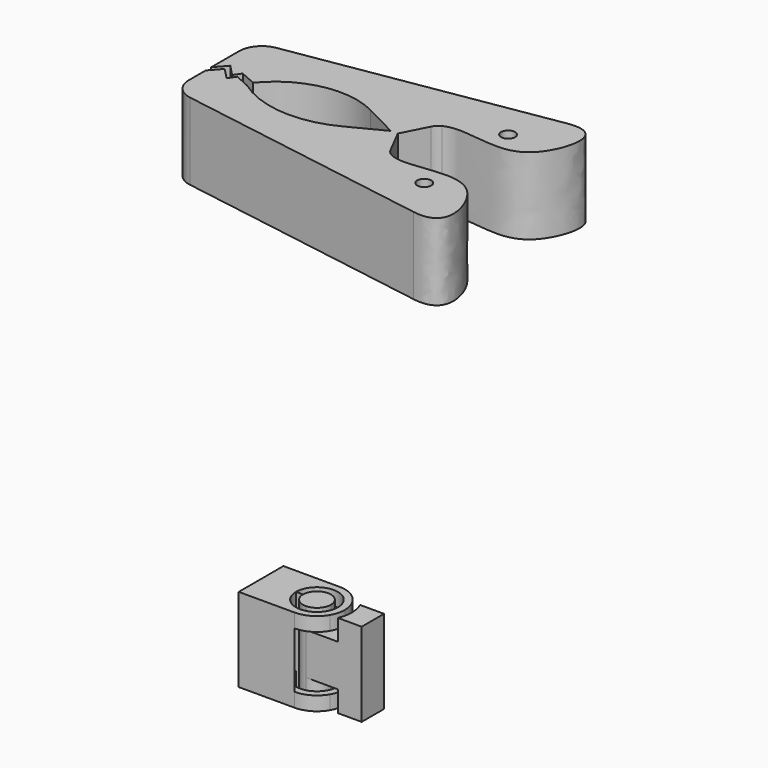
from build123d import *

# Parameters (mm, degrees)
F0_R     = 1
F1_DEPTH = 11
F3_DEPTH = 6
F4_DEPTH = 4
F5_DEPTH = 3
F6_DEPTH = 6


# Not quite as in the source:
# - a feature names something its author has since deleted; it is built from what else it names


with BuildPart() as f1:
    # F0 (on Top) → F1 (new body)
    with BuildSketch(Plane.XY):
        with BuildLine():
            Line((-56.5394303022, 63.5646519078), (-56.5394303022, 60.5646519078))
            Line((-56.5394303022, 60.5646519078), (-56.5394303022, 58.5646519078))
            Line((-56.5394303022, 58.5646519078), (-55.1112962965, 60.1865433678))
            Line((-55.1112962965, 60.1865433678), (-53.5394303022, 58.5646519078))
            Line((-53.5394303022, 58.5646519078), (-52.8413255975, 59.585552632))
            Line((-52.8413255975, 59.585552632), (-50.5394303022, 58.5646519078))
            ThreePointArc((-50.5394303022, 58.5646519078), (-43.8778670045, 62.6266002152), (-36.1451600741, 61.5868439218))
            Line((-36.1451600741, 61.5868439218), (-31.2319873402, 59.0646519078))
            Line((-31.2319873402, 59.0646519078), (-36.1451600741, 56.5424598938))
            ThreePointArc((-36.1451600741, 56.5424598938), (-43.5460973086, 55.0399418647), (-50.6461998164, 57.612873414))
            Line((-50.6461998164, 57.612873414), (-52.831540008, 58.5998629716))
            Line((-52.831540008, 58.5998629716), (-53.5394303022, 57.5646519078))
            Line((-53.5394303022, 57.5646519078), (-55.1112962965, 59.1865433678))
            Line((-55.1112962965, 59.1865433678), (-56.5394303022, 57.5646519078))
            Line((-56.5394303022, 57.5646519078), (-56.5394303022, 54.5646519078))
            ThreePointArc((-56.5394303022, 54.5646519078), (-55.7660672354, 52.4605684374), (-53.8141510367, 51.3581706702))
            Line((-53.8141510367, 51.3581706702), (-17.0027786636, 45.3461106944))
            add(Edge.make_bspline(
                [(-27.5149940739, 54.5646519078), (-25.8077646027, 53.6646211006), (-20.1492133777, 55.1651591419), (-13.9447941806, 53.7805000119), (-11.9302922568, 44.5176685435), (-17.0027786636, 45.3461106944)],
                knots=[0, 0, 0, 0, 0.3389884786, 0.6657804562, 1, 1, 1, 1], degree=3))
            ThreePointArc((-27.5149940739, 54.5646519078), (-28.0042315995, 54.9274057779), (-28.3616043344, 55.4205877474))
            Line((-28.3616043344, 55.4205877474), (-30.2319873402, 59.0646519078))
            Line((-30.2319873402, 59.0646519078), (-28.3616043344, 62.7087160682))
            ThreePointArc((-28.3616043344, 62.7087160682), (-28.0042315995, 63.2018980376), (-27.5149940739, 63.5646519078))
            add(Edge.make_bspline(
                [(-27.5149940739, 63.5646519078), (-25.8077646027, 64.464682715), (-20.1492133777, 62.9641446737), (-13.9447941806, 64.3488038037), (-11.9302922568, 73.6116352721), (-17.0027786636, 72.7831931212)],
                knots=[0, 0, 0, 0, 0.3389884786, 0.6657804562, 1, 1, 1, 1], degree=3))
            Line((-17.0027786636, 72.7831931212), (-53.8141510367, 66.7711331454))
            ThreePointArc((-53.8141510367, 66.7711331454), (-55.7660672354, 65.6687353782), (-56.5394303022, 63.5646519078))
        make_face()
        with Locations((-20.4416182045, 51.5646519078)):
            Circle(F0_R, mode=Mode.SUBTRACT)
        with Locations((-20.4416182045, 66.5646519078)):
            Circle(F0_R, mode=Mode.SUBTRACT)
    extrude(amount=F1_DEPTH)


with BuildPart() as f3:
    # F2 (on Top) → F3 (new body, symmetric)
    with BuildSketch(Plane.XY):
        with BuildLine():
            ThreePointArc((27.1985391751, -29.1886593086), (28.6127527375, -28.602872871), (29.1985391751, -27.1886593086))
            ThreePointArc((29.1985391751, -27.1886593086), (28.6127527375, -25.7744457462), (27.1985391751, -25.1886593086))
            ThreePointArc((27.1985391751, -25.1886593086), (25.7846792103, -25.774092237), (25.1985394251, -27.1876593086))
            ThreePointArc((25.1985394251, -27.1876593086), (25.1985391751, -27.1886593086), (25.1985394251, -27.1896593086))
            ThreePointArc((25.1985394251, -27.1896593086), (25.7846792103, -28.6032263802), (27.1985391751, -29.1886593086))
        make_face()
        with BuildLine():
            ThreePointArc((25.1985394251, -27.1896593086), (25.1985391751, -27.1886593086), (25.1985394251, -27.1876593086))
            Line((25.1985394251, -27.1876593086), (24.1985393418, -27.1876593086))
            ThreePointArc((24.1985393418, -27.1876593086), (24.1985391751, -27.1886593086), (24.1985393418, -27.1896593086))
            Line((24.1985393418, -27.1896593086), (25.1985394251, -27.1896593086))
        make_face()
        with BuildLine():
            Line((30.6626407902, -25.1886593086), (29.4346071526, -25.1886593086))
            ThreePointArc((29.4346071526, -25.1886593086), (30.001056252, -26.1181930393), (30.1985391751, -27.1886593086))
            ThreePointArc((30.1985391751, -27.1886593086), (30.001056252, -28.2591255779), (29.4346071526, -29.1886593086))
            Line((29.4346071526, -29.1886593086), (30.6626407902, -29.1886593086))
            ThreePointArc((30.6626407902, -29.1886593086), (31.0622424802, -28.223935489), (31.1985391751, -27.1886593086))
            ThreePointArc((31.1985391751, -27.1886593086), (31.0622424802, -26.1533831282), (30.6626407902, -25.1886593086))
        make_face()
        with BuildLine():
            ThreePointArc((24.1985393418, -27.1876593086), (26.1285400068, -24.3859638596), (29.4346071526, -25.1886593086))
            Line((29.4346071526, -25.1886593086), (30.6626407902, -25.1886593086))
            ThreePointArc((30.6626407902, -25.1886593086), (29.1985391751, -23.7245576935), (27.1985391751, -23.1886593086))
            ThreePointArc((27.1985391751, -23.1886593086), (24.3704656258, -24.3598786525), (23.1985393001, -27.1876593086))
            Line((23.1985393001, -27.1876593086), (24.1985393418, -27.1876593086))
        make_face()
        with BuildLine():
            Line((30.6626407902, -29.1886593086), (29.4346071526, -29.1886593086))
            ThreePointArc((29.4346071526, -29.1886593086), (26.1285400068, -29.9913547576), (24.1985393418, -27.1896593086))
            Line((24.1985393418, -27.1896593086), (23.1985393001, -27.1896593086))
            ThreePointArc((23.1985393001, -27.1896593086), (24.3704656258, -30.0174399646), (27.1985391751, -31.1886593086))
            ThreePointArc((27.1985391751, -31.1886593086), (29.1985391751, -30.6527609237), (30.6626407902, -29.1886593086))
        make_face()
        with BuildLine():
            ThreePointArc((24.1985393418, -27.1896593086), (24.1985391751, -27.1886593086), (24.1985393418, -27.1876593086))
            Line((24.1985393418, -27.1876593086), (23.1985393001, -27.1876593086))
            ThreePointArc((23.1985393001, -27.1876593086), (23.1985391751, -27.1886593086), (23.1985393001, -27.1896593086))
            Line((23.1985393001, -27.1896593086), (24.1985393418, -27.1896593086))
        make_face()
        with BuildLine():
            ThreePointArc((23.1985393001, -27.1896593086), (23.1985391751, -27.1886593086), (23.1985393001, -27.1876593086))
            ThreePointArc((23.1985393001, -27.1876593086), (24.3704656258, -24.3598786525), (27.1985391751, -23.1886593086))
            Line((27.1985391751, -23.1886593086), (24.1985391751, -23.1886593086))
            ThreePointArc((24.1985391751, -23.1886593086), (22.1985391751, -27.1886593086), (24.1985391751, -31.1886593086))
            Line((24.1985391751, -31.1886593086), (27.1985391751, -31.1886593086))
            ThreePointArc((27.1985391751, -31.1886593086), (24.3704656258, -30.0174399646), (23.1985393001, -27.1896593086))
        make_face()
        with BuildLine():
            ThreePointArc((24.1985391751, -31.1886593086), (22.1985391751, -27.1886593086), (24.1985391751, -23.1886593086))
            Line((24.1985391751, -23.1886593086), (19.1985391751, -23.1886593086))
            Line((19.1985391751, -23.1886593086), (19.1985391751, -31.1886593086))
            Line((19.1985391751, -31.1886593086), (24.1985391751, -31.1886593086))
        make_face()
    extrude(amount=F3_DEPTH, both=True)

    # F2 (on Top) → F4 (cut, symmetric)
    with BuildSketch(Plane.XY):
        with BuildLine():
            ThreePointArc((24.1985393418, -27.1876593086), (26.1285400068, -24.3859638596), (29.4346071526, -25.1886593086))
            Line((29.4346071526, -25.1886593086), (30.6626407902, -25.1886593086))
            ThreePointArc((30.6626407902, -25.1886593086), (29.1985391751, -23.7245576935), (27.1985391751, -23.1886593086))
            ThreePointArc((27.1985391751, -23.1886593086), (24.3704656258, -24.3598786525), (23.1985393001, -27.1876593086))
            Line((23.1985393001, -27.1876593086), (24.1985393418, -27.1876593086))
        make_face()
        with BuildLine():
            Line((30.6626407902, -25.1886593086), (29.4346071526, -25.1886593086))
            ThreePointArc((29.4346071526, -25.1886593086), (30.001056252, -26.1181930393), (30.1985391751, -27.1886593086))
            ThreePointArc((30.1985391751, -27.1886593086), (30.001056252, -28.2591255779), (29.4346071526, -29.1886593086))
            Line((29.4346071526, -29.1886593086), (30.6626407902, -29.1886593086))
            ThreePointArc((30.6626407902, -29.1886593086), (31.0622424802, -28.223935489), (31.1985391751, -27.1886593086))
            ThreePointArc((31.1985391751, -27.1886593086), (31.0622424802, -26.1533831282), (30.6626407902, -25.1886593086))
        make_face()
        with BuildLine():
            Line((30.6626407902, -29.1886593086), (29.4346071526, -29.1886593086))
            ThreePointArc((29.4346071526, -29.1886593086), (26.1285400068, -29.9913547576), (24.1985393418, -27.1896593086))
            Line((24.1985393418, -27.1896593086), (23.1985393001, -27.1896593086))
            ThreePointArc((23.1985393001, -27.1896593086), (24.3704656258, -30.0174399646), (27.1985391751, -31.1886593086))
            ThreePointArc((27.1985391751, -31.1886593086), (29.1985391751, -30.6527609237), (30.6626407902, -29.1886593086))
        make_face()
    extrude(amount=F4_DEPTH, both=True, mode=Mode.SUBTRACT)

    # F2 (on Top) → F5 (join, symmetric)
    with BuildSketch(Plane.XY):
        with BuildLine():
            ThreePointArc((27.1985391751, -25.1886593086), (28.6127527375, -25.7744457462), (29.1985391751, -27.1886593086))
            ThreePointArc((29.1985391751, -27.1886593086), (28.6127527375, -28.602872871), (27.1985391751, -29.1886593086))
            Line((27.1985391751, -29.1886593086), (29.4346071526, -29.1886593086))
            ThreePointArc((29.4346071526, -29.1886593086), (30.001056252, -28.2591255779), (30.1985391751, -27.1886593086))
            ThreePointArc((30.1985391751, -27.1886593086), (30.001056252, -26.1181930393), (29.4346071526, -25.1886593086))
            Line((29.4346071526, -25.1886593086), (27.1985391751, -25.1886593086))
        make_face()
        with BuildLine():
            Line((31.78111487, -25.1886593086), (30.6626407902, -25.1886593086))
            ThreePointArc((30.6626407902, -25.1886593086), (31.0622424802, -26.1533831282), (31.1985391751, -27.1886593086))
            ThreePointArc((31.1985391751, -27.1886593086), (31.0622424802, -28.223935489), (30.6626407902, -29.1886593086))
            Line((30.6626407902, -29.1886593086), (31.78111487, -29.1886593086))
            ThreePointArc((31.78111487, -29.1886593086), (32.0930707397, -28.210207527), (32.1985391751, -27.1886593086))
            ThreePointArc((32.1985391751, -27.1886593086), (32.0930707397, -26.1671110901), (31.78111487, -25.1886593086))
        make_face()
        with BuildLine():
            Line((30.6626407902, -25.1886593086), (29.4346071526, -25.1886593086))
            ThreePointArc((29.4346071526, -25.1886593086), (30.001056252, -26.1181930393), (30.1985391751, -27.1886593086))
            ThreePointArc((30.1985391751, -27.1886593086), (30.001056252, -28.2591255779), (29.4346071526, -29.1886593086))
            Line((29.4346071526, -29.1886593086), (30.6626407902, -29.1886593086))
            ThreePointArc((30.6626407902, -29.1886593086), (31.0622424802, -28.223935489), (31.1985391751, -27.1886593086))
            ThreePointArc((31.1985391751, -27.1886593086), (31.0622424802, -26.1533831282), (30.6626407902, -25.1886593086))
        make_face()
    extrude(amount=F5_DEPTH, both=True)

    # F2 (on Top) → F6 (join, symmetric)
    with BuildSketch(Plane.XY):
        with BuildLine():
            Line((35.1985391751, -25.1886593086), (31.78111487, -25.1886593086))
            ThreePointArc((31.78111487, -25.1886593086), (32.0930707397, -26.1671110901), (32.1985391751, -27.1886593086))
            ThreePointArc((32.1985391751, -27.1886593086), (32.0930707397, -28.210207527), (31.78111487, -29.1886593086))
            Line((31.78111487, -29.1886593086), (35.1985391751, -29.1886593086))
            Line((35.1985391751, -29.1886593086), (35.1985391751, -25.1886593086))
        make_face()
    extrude(amount=F6_DEPTH, both=True)


solid = Compound([f1.part, f3.part])
